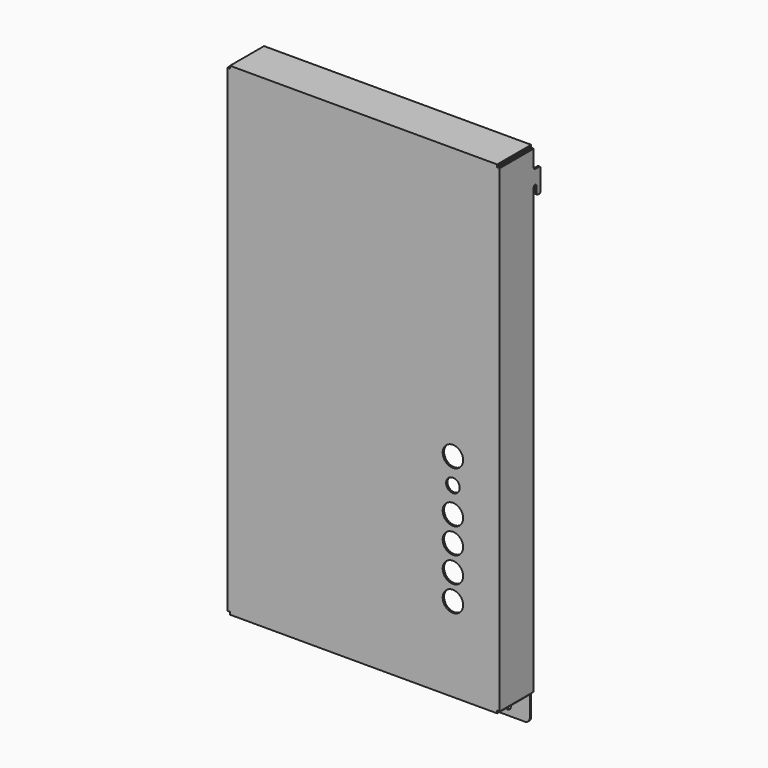
from build123d import *

# Parameters (mm, degrees)
F0_W      = 160
F0_H      = 284
F1_DEPTH  = 1
F2_W      = 160
F2_H      = 284
F2_W_2    = 158
F2_H_2    = 282
F3_DEPTH  = 24
F4_W      = 1.5
F4_H      = 1.5
F5_DEPTH  = 25.001
F6_R      = 6
F6_R_2    = 4
F7_DEPTH  = 25.001
F8_W      = 157
F8_H      = 1
F9_DEPTH  = 15
F10_R     = 3
F12_DEPTH = 1.001
F13_W     = 1
F13_H     = 8
F14_DEPTH = 5
F15_W     = 1
F15_H     = 3
F16_DEPTH = 6
F17_R     = 0.99999
F18_R     = 0.99999


# Not quite as in the source:
# - a fillet or chamfer is up to 0.001 mm smaller than in the source, because OpenCascade refuses the exact size


with BuildPart() as f1:
    # F0 (on Front) → F1 (new body)
    with BuildSketch(Plane.XZ):
        with Locations((80, 142)):
            Rectangle(F0_W, F0_H)
    extrude(amount=F1_DEPTH)

    # F2 (on face) → F3 (join)
    with BuildSketch(Plane(origin=(0, 0, 0), x_dir=(-1, 0, 0), z_dir=(0, 1, 0))):
        with Locations((-80, 142)):
            Rectangle(F2_W, F2_H)
        with Locations((-80, 142)):
            Rectangle(F2_W_2, F2_H_2, mode=Mode.SUBTRACT)
    extrude(amount=F3_DEPTH)

    # F4 (on face) → F5 (cut, through all)
    with BuildSketch(Plane.XZ.offset(1)):
        with Locations((0.75, 283.25)):
            Rectangle(F4_W, F4_H)
        with Locations((159.25, 283.25)):
            Rectangle(F4_W, F4_H)
        with Locations((159.25, 0.75)):
            Rectangle(F4_W, F4_H)
        with Locations((0.75, 0.75)):
            Rectangle(F4_W, F4_H)
    extrude(amount=-F5_DEPTH, mode=Mode.SUBTRACT)

    # F6 (on face) → F7 (cut, through all)
    with BuildSketch(Plane.XZ.offset(1)):
        with Locations((132.5, 124.5)):
            Circle(F6_R)
        with Locations((132.5, 109.5)):
            Circle(F6_R_2)
        with Locations((132.5, 94.5)):
            Circle(F6_R)
        with Locations((132.5, 79.5)):
            Circle(F6_R)
        with Locations((132.5, 64.5)):
            Circle(F6_R)
        with Locations((132.5, 49.5)):
            Circle(F6_R)
    extrude(amount=-F7_DEPTH, mode=Mode.SUBTRACT)

    # F8 (on face) → F9 (join)
    with BuildSketch(Plane(origin=(0, 0, 0), x_dir=(1, 0, 0), z_dir=(0, 0, -1))):
        with Locations((80, -23.5)):
            Rectangle(F8_W, F8_H)
    extrude(amount=F9_DEPTH)

    # F10
    f10_edges = [f1.edges().sort_by_distance(p)[0] for p in [
        (1.5, 23.5, -15),
        (158.5, 23.5, -15),
    ]]
    fillet(f10_edges, radius=F10_R)

    # F11 (on face) → F12 (cut, through all)
    with BuildSketch(Plane.XZ.offset(-23)):
        with BuildLine():
            ThreePointArc((16.3, -7.8), (14.5, -6), (12.7, -7.8))
            Line((12.7, -7.8), (12.7, -10.2))
            ThreePointArc((12.7, -10.2), (14.5, -12), (16.3, -10.2))
            Line((16.3, -10.2), (16.3, -7.8))
        make_face()
        with BuildLine():
            ThreePointArc((147.3, -7.8), (145.5, -6), (143.7, -7.8))
            Line((143.7, -7.8), (143.7, -10.2))
            ThreePointArc((143.7, -10.2), (145.5, -12), (147.3, -10.2))
            Line((147.3, -10.2), (147.3, -7.8))
        make_face()
    extrude(amount=-F12_DEPTH, mode=Mode.SUBTRACT)

    # F13 (on face) → F14 (join)
    with BuildSketch(Plane(origin=(0, 24, 0), x_dir=(-1, 0, 0), z_dir=(0, 1, 0))):
        with Locations((-159.5, 267.5)):
            Rectangle(F13_W, F13_H)
        with Locations((-0.5, 267.5)):
            Rectangle(F13_W, F13_H)
    extrude(amount=F14_DEPTH)

    # F15 (on face) → F16 (join)
    with BuildSketch(Plane(origin=(0, 0, 263.5), x_dir=(1, 0, 0), z_dir=(0, 0, -1))):
        with Locations((159.5, -27.5)):
            Rectangle(F15_W, F15_H)
        with Locations((0.5, -27.5)):
            Rectangle(F15_W, F15_H)
    extrude(amount=F16_DEPTH)

    # F17 (radius 1 in the source; OpenCascade refuses exactly that, so slightly less here)
    f17_edges = [f1.edges().sort_by_distance(p)[0] for p in [
        (0.5, 26, 263.5),
        (0.5, 26, 257.5),
        (0.5, 29, 257.5),
        (0.5, 24, 263.5),
        (0.5, 24, 271.5),
        (0.5, 29, 271.5),
    ]]
    fillet(f17_edges, radius=F17_R)

    # F18 (radius 1 in the source; OpenCascade refuses exactly that, so slightly less here)
    f18_edges = [f1.edges().sort_by_distance(p)[0] for p in [
        (159.5, 24, 271.5),
        (159.5, 29, 271.5),
        (159.5, 29, 257.5),
        (159.5, 24, 263.5),
        (159.5, 26, 257.5),
        (159.5, 26, 263.5),
    ]]
    fillet(f18_edges, radius=F18_R)


solid = f1.part
